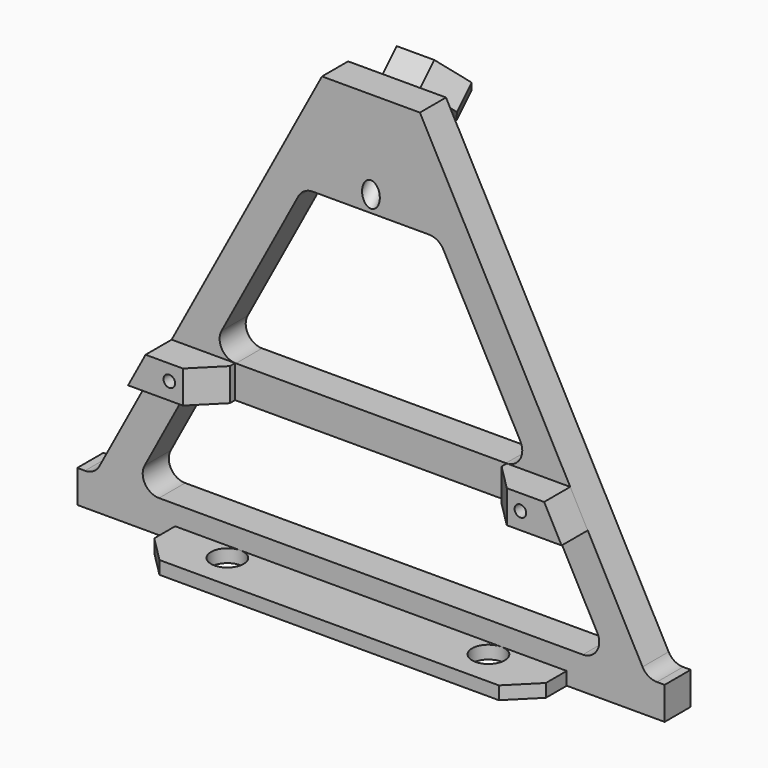
from build123d import *

# Parameters (mm, degrees)
F1_DEPTH  = 6.35
F2_R      = 3.175
F3_W      = 76.2
F3_H      = 2.54
F4_DEPTH  = 10.16
F5_SIZE   = 5.08
F7_DEPTH  = 6.35
F8_SIZE   = 5.08
F10_D     = 2.2606
F13_DEPTH = 5.08
F14_R     = 5.3951847675
F15_REACH = 89.7970127444
F17_D     = 3.4544
F19_D     = 6.35
F19_DEPTH = 2.541


with BuildPart() as f1:
    # F0 (on Front) → F1 (new body)
    with BuildSketch(Plane.XZ):
        Polygon((9.525, 88.9), (-9.525, 88.9), (-53.7482142857, 6.35), (-57.15, 0), (57.15, 0), (53.7482142857, 6.35), align=None)
        with BuildLine():
            Line((41.2416306314, 6.35), (-41.2416306314, 6.35))
            ThreePointArc((-41.2416306314, 6.35), (-43.9656820238, 7.8939975439), (-44.0403295363, 11.0243029847))
            Line((-44.0403295363, 11.0243029847), (-35.876043822, 26.2643029847))
            ThreePointArc((-35.876043822, 26.2643029847), (-34.7083473732, 27.4890513924), (-33.0773449171, 27.94))
            Line((-33.0773449171, 27.94), (33.0773449171, 27.94))
            ThreePointArc((33.0773449171, 27.94), (34.7083473732, 27.4890513924), (35.876043822, 26.2643029847))
            Line((35.876043822, 26.2643029847), (44.0403295363, 11.0243029847))
            ThreePointArc((44.0403295363, 11.0243029847), (43.9656820238, 7.8939975439), (41.2416306314, 6.35))
        make_face(mode=Mode.SUBTRACT)
        with BuildLine():
            ThreePointArc((-14.1046152506, 66.9043029847), (-12.9369188018, 68.1290513924), (-11.3059163457, 68.58))
            Line((-11.3059163457, 68.58), (11.3059163457, 68.58))
            ThreePointArc((11.3059163457, 68.58), (12.9369188018, 68.1290513924), (14.1046152506, 66.9043029847))
            Line((14.1046152506, 66.9043029847), (29.0724723934, 38.9643029847))
            ThreePointArc((29.0724723934, 38.9643029847), (28.9978248809, 35.8339975439), (26.2737734886, 34.29))
            Line((26.2737734886, 34.29), (-26.2737734886, 34.29))
            ThreePointArc((-26.2737734886, 34.29), (-28.9978248809, 35.8339975439), (-29.0724723934, 38.9643029847))
            Line((-29.0724723934, 38.9643029847), (-14.1046152506, 66.9043029847))
        make_face(mode=Mode.SUBTRACT)
        Polygon((-57.15, 0), (-53.7482142857, 6.35), (-57.15, 6.35), align=None)
        Polygon((57.15, 6.35), (53.7482142857, 6.35), (57.15, 0), align=None)
    extrude(amount=F1_DEPTH)

    # F2
    f2_edges = [f1.edges().sort_by_distance(p)[0] for p in [
        (53.748214, -3.175, 6.35),
        (-53.748214, -3.175, 6.35),
    ]]
    fillet(f2_edges, radius=F2_R)

    # F3 (on face) → F4 (join)
    with BuildSketch(Plane.XZ.offset(6.35)):
        with Locations((0, 1.27)):
            Rectangle(F3_W, F3_H)
    extrude(amount=F4_DEPTH)

    # F5
    f5_edges = [f1.edges().sort_by_distance(p)[0] for p in [
        (-38.1, -16.51, 1.27),
        (38.1, -16.51, 1.27),
    ]]
    chamfer(f5_edges, length=F5_SIZE)

    # F6 (on face) → F7 (join)
    with BuildSketch(Plane.XZ.offset(6.35)):
        Polygon((-42.1821428571, 27.94), (-33.0773449171, 27.94), (-26.4341428571, 27.94), (-26.4341428571, 34.29), (-38.7803571429, 34.29), align=None)
        Polygon((26.4341428571, 34.29), (26.4341428571, 27.94), (33.0773449171, 27.94), (42.1821428571, 27.94), (38.7803571429, 34.29), align=None)
    extrude(amount=F7_DEPTH)

    # F8
    f8_edges = [f1.edges().sort_by_distance(p)[0] for p in [
        (26.434143, -12.7, 31.115),
        (-26.434143, -12.7, 31.115),
    ]]
    chamfer(f8_edges, length=F8_SIZE)

    # F10 (through all)
    with Locations(Plane.XZ.offset(12.7)):
        with Locations((-34.163, 31.242), (34.163, 31.242)):
            Hole(F10_D / 2)



with BuildPart() as f13:
    # F12 (on face) → F13 (new body)
    with BuildSketch(Plane(origin=(0, 44.45, 44.45), x_dir=(-1, 0, 0), z_dir=(0, 0.7071067812, 0.7071067812))):
        Polygon((-3.6661742094, 48.8917928475), (3.6661742094, 48.8917928475), (7.3323484187, 55.2417928475), (3.6661742094, 61.5917928475), (-3.6661742094, 61.5917928475), (-7.3323484187, 55.2417928475), align=None)
    extrude(amount=F13_DEPTH)


with BuildPart() as f1_1:
    add(f1.part)

    add(f13.part)  # F15 merges F13
    f15_end = f1_1.faces().sort_by_distance((-29.9113566426, 0, 47.7790611404))[0]
    # F14 (on face) → F15 (join, up to a face of the model that its end follows)
    with BuildSketch(Plane(origin=(0, 44.45, 44.45), x_dir=(1, 0, 0), z_dir=(0, -0.7071067812, -0.7071067812))):
        with Locations((0, 55.2417928475)):
            Circle(F14_R)
    f15_long = extrude(amount=F15_REACH, mode=Mode.PRIVATE)
    add(split(f15_long, bisect_by=f15_end, keep=Keep.TOP, mode=Mode.PRIVATE))

    # F17 (through all)
    with Locations(Plane(origin=(0, 48.0421024484, 48.0421024484), x_dir=(-1, 0, 0), z_dir=(0, 0.7071067812, 0.7071067812))):
        with Locations((0, 55.2417928475)):
            Hole(F17_D / 2)

    # F19 (through all, one way)
    with BuildSketch(Plane.XY.offset(2.54)):
        with Locations((-25.4, -9.525), (25.4, -9.525)):
            Circle(F19_D / 2)
    extrude(amount=-F19_DEPTH, mode=Mode.SUBTRACT)


solid = f1_1.part
